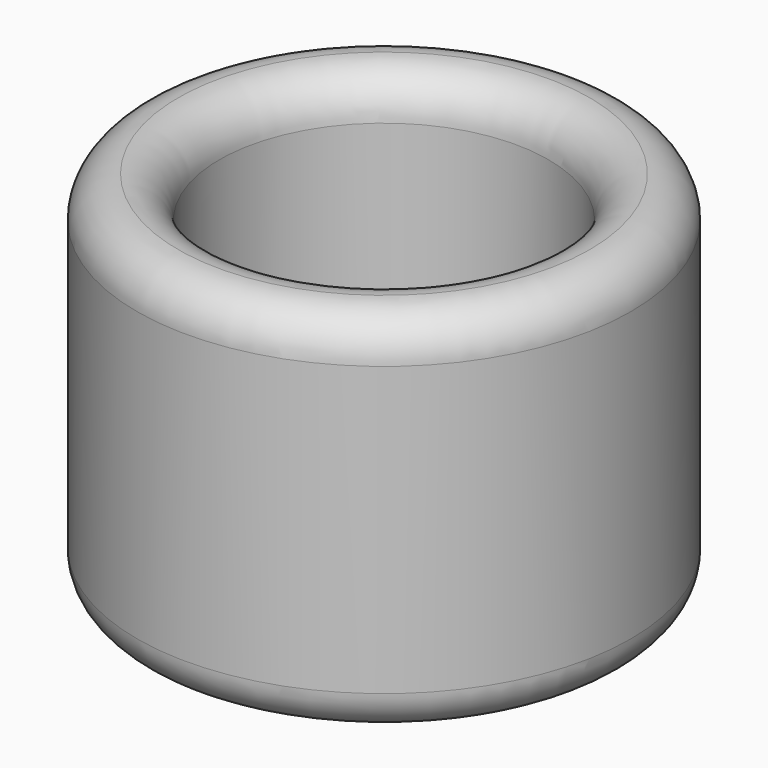
from build123d import *

# Parameters (mm, degrees)
F0_R     = 30
F0_R_2   = 20
F1_DEPTH = 45
F2_R     = 4.99999


# Not quite as in the source:
# - a fillet or chamfer is up to 0.001 mm smaller than in the source, because OpenCascade refuses the exact size


with BuildPart() as f1:
    # F0 (on Top) → F1 (new body)
    with BuildSketch(Plane.XY):
        with Locations((0, -1.9317325205)):
            Circle(F0_R)
        with Locations((0, -1.9317325205)):
            Circle(F0_R_2, mode=Mode.SUBTRACT)
    extrude(amount=F1_DEPTH)

    # F2 (radius 5 in the source; OpenCascade refuses exactly that, so slightly less here)
    f2_edges = [f1.edges().sort_by_distance(p)[0] for p in [
        (-30, -1.931733, 0),
        (-20, -1.931733, 0),
        (-20, -1.931733, 45),
        (-30, -1.931733, 45),
    ]]
    fillet(f2_edges, radius=F2_R)


solid = f1.part
